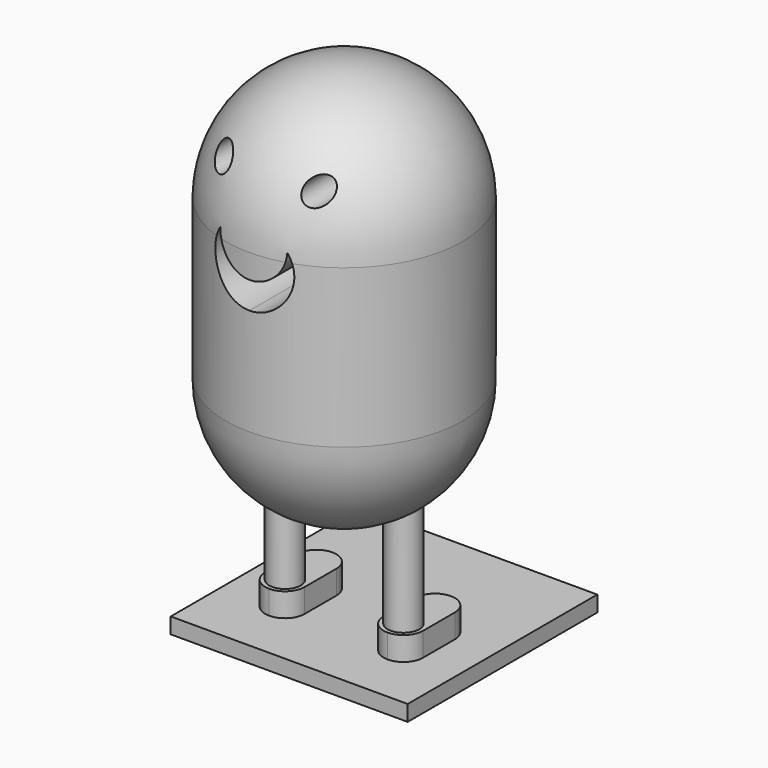
from build123d import *

# Parameters (mm, degrees)
F0_W     = 30
F0_H     = 30
F1_DEPTH = 2
F0_R     = 2
F3_DEPTH = 5
F4_DEPTH = 25
F2_R     = 1.5
F6_DEPTH = 15
F7_DEPTH = 15


# Not quite as in the source:
# - a feature names something its author has since deleted; it is built from what else it names


with BuildPart() as f1:
    # F0 (on Top) → F1 (new body)
    with BuildSketch(Plane.XY):
        with Locations((0, 6.2995284576)):
            Rectangle(F0_W, F0_H)
        with BuildLine():
            ThreePointArc((-10, 5), (-9.267766953, 6.767766953), (-7.5, 7.5))
            ThreePointArc((-7.5, 7.5), (-5.732233047, 6.767766953), (-5, 5))
            Line((-5, 5), (-5, 0))
            ThreePointArc((-5, 0), (-5.732233047, -1.767766953), (-7.5, -2.5))
            ThreePointArc((-7.5, -2.5), (-9.267766953, -1.767766953), (-10, 0))
            Line((-10, 0), (-10, 5))
        make_face(mode=Mode.SUBTRACT)
        with BuildLine():
            Line((5, 0), (5, 5))
            ThreePointArc((5, 5), (5.732233047, 6.767766953), (7.5, 7.5))
            ThreePointArc((7.5, 7.5), (9.267766953, 6.767766953), (10, 5))
            Line((10, 5), (10, 0))
            ThreePointArc((10, 0), (9.267766953, -1.767766953), (7.5, -2.5))
            ThreePointArc((7.5, -2.5), (5.732233047, -1.767766953), (5, 0))
        make_face(mode=Mode.SUBTRACT)
    extrude(amount=F1_DEPTH)

    # F0 (on Top) → F3 (join)
    with BuildSketch(Plane.XY):
        with BuildLine():
            ThreePointArc((7.5, 7.5), (5.732233047, 6.767766953), (5, 5))
            Line((5, 5), (5, 0))
            ThreePointArc((5, 0), (5.732233047, -1.767766953), (7.5, -2.5))
            ThreePointArc((7.5, -2.5), (9.267766953, -1.767766953), (10, 0))
            Line((10, 0), (10, 5))
            ThreePointArc((10, 5), (9.267766953, 6.767766953), (7.5, 7.5))
        make_face()
        with Locations((7.5, 0)):
            Circle(F0_R, mode=Mode.SUBTRACT)
        with BuildLine():
            ThreePointArc((-5, 5), (-5.732233047, 6.767766953), (-7.5, 7.5))
            ThreePointArc((-7.5, 7.5), (-9.267766953, 6.767766953), (-10, 5))
            Line((-10, 5), (-10, 0))
            ThreePointArc((-10, 0), (-9.267766953, -1.767766953), (-7.5, -2.5))
            ThreePointArc((-7.5, -2.5), (-5.732233047, -1.767766953), (-5, 0))
            Line((-5, 0), (-5, 5))
        make_face()
        with Locations((-7.5, 0)):
            Circle(F0_R, mode=Mode.SUBTRACT)
    extrude(amount=F3_DEPTH)

    # F0 (on Top) → F4 (join)
    with BuildSketch(Plane.XY):
        with Locations((7.5, 0)):
            Circle(F0_R)
        with Locations((-7.5, 0)):
            Circle(F0_R)
    extrude(amount=F4_DEPTH)

    # F2 (on Front) → F5 (revolve)
    with BuildSketch(Plane.XZ):
        with BuildLine():
            ThreePointArc((15, 50), (10.6066017178, 60.6066017178), (0, 65))
            Line((0, 65), (0, 46.9528951543))
            ThreePointArc((0, 46.9528951543), (3.0017193367, 48.1526751529), (4.2698885231, 51.1261475231))
            ThreePointArc((4.2698885231, 51.1261475231), (4.3593428406, 46.0758998678), (0, 43.5245995224))
            Line((0, 43.5245995224), (0, 15))
            ThreePointArc((0, 15), (10.6066017178, 19.3933982822), (15, 30))
            Line((15, 30), (15, 50))
        make_face()
        with Locations((6, 57.3495886624)):
            Circle(F2_R, mode=Mode.SUBTRACT)
        with Locations((6, 57.3495886624)):
            Circle(F2_R)
        with BuildLine():
            ThreePointArc((4.2698885231, 51.1261475231), (3.0017193367, 48.1526751529), (0, 46.9528951543))
            Line((0, 46.9528951543), (0, 43.5245995224))
            ThreePointArc((0, 43.5245995224), (4.3593428406, 46.0758998678), (4.2698885231, 51.1261475231))
        make_face()
    revolve(axis=Axis((0, 0, 40), (0, 0, -1)))

    # F2 (on Front) → F6 (cut, symmetric)
    with BuildSketch(Plane.XZ):
        with Locations((6, 57.3495886624)):
            Circle(F2_R)
        with Locations((-6, 57.3495886624)):
            Circle(F2_R)
    extrude(amount=F6_DEPTH, both=True, mode=Mode.SUBTRACT)

    # F2 (on Front) → F7 (cut, symmetric)
    with BuildSketch(Plane.XZ):
        with BuildLine():
            ThreePointArc((4.2698885231, 51.1261475231), (3.0017193367, 48.1526751529), (0, 46.9528951543))
            Line((0, 46.9528951543), (0, 43.5245995224))
            ThreePointArc((0, 43.5245995224), (4.3593428406, 46.0758998678), (4.2698885231, 51.1261475231))
        make_face()
        with BuildLine():
            Line((0, 43.5245995224), (0, 46.9528951543))
            ThreePointArc((0, 46.9528951543), (-2.9917232596, 48.2573678623), (-4.1542744288, 51.3070452037))
            ThreePointArc((-4.1542744288, 51.3070452037), (-4.4109085463, 46.1700537495), (0, 43.5245995224))
        make_face()
    extrude(amount=F7_DEPTH, both=True, mode=Mode.SUBTRACT)


solid = f1.part
